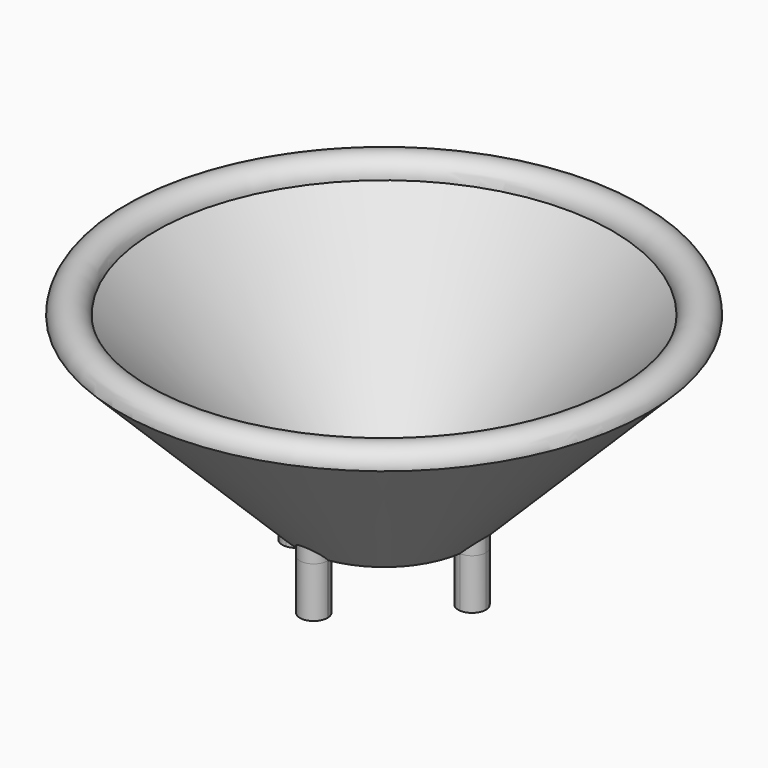
from build123d import *
from build123d import SkipClean  # not in build123d's __all__

# Parameters (mm, degrees)
F4_DEPTH = 10


with BuildPart() as f1:
    # F0 (on Front) → F1 (revolve)
    with BuildSketch(Plane.XZ):
        with BuildLine():
            Line((0, 5), (0, 0))
            Line((0, 0), (17.5, 0))
            Line((17.5, 0), (48.9644660941, 31.4644660941))
            ThreePointArc((48.9644660941, 31.4644660941), (46.4644660941, 32.5), (45.4289321881, 35))
            Line((45.4289321881, 35), (15.4289321881, 5))
            Line((15.4289321881, 5), (0, 5))
        make_face()
        with BuildLine():
            Line((45.4289321881, 35), (52.5, 35))
            ThreePointArc((52.5, 35), (48.9644660941, 38.5355339059), (45.4289321881, 35))
        make_face()
        with BuildLine():
            ThreePointArc((45.4289321881, 35), (46.4644660941, 32.5), (48.9644660941, 31.4644660941))
            Line((48.9644660941, 31.4644660941), (52.5, 35))
            Line((52.5, 35), (45.4289321881, 35))
        make_face()
    revolve(axis=Axis((0, 0, 17.5), (0, 0, 1)))

    # F2 (on face) → F3 (join, up to the next surface of F1)
    with BuildSketch(Plane(origin=(0, 0, 0), x_dir=(1, 0, 0), z_dir=(0, 0, -1))):
        with BuildLine():
            ThreePointArc((17.2839285714, -2.7414983381), (19.3665882743, -2.0194920684), (20.25, 0))
            ThreePointArc((20.25, 0), (19.3665882743, 2.0194920684), (17.2839285714, 2.7414983381))
            ThreePointArc((17.2839285714, 2.7414983381), (17.4458985151, 1.375), (17.5, 0))
            ThreePointArc((17.5, 0), (17.4458985151, -1.375), (17.2839285714, -2.7414983381))
        make_face()
        with BuildLine():
            ThreePointArc((-2.7414983381, 17.2839285714), (0, 17.5), (2.7414983381, 17.2839285714))
            ThreePointArc((2.7414983381, 17.2839285714), (2.7478737625, 17.3918806903), (2.75, 17.5))
            ThreePointArc((2.75, 17.5), (-0.1081193097, 20.2478737625), (-2.7414983381, 17.2839285714))
        make_face()
        with BuildLine():
            ThreePointArc((-2.7414983381, 17.2839285714), (0, 14.75), (2.7414983381, 17.2839285714))
            ThreePointArc((2.7414983381, 17.2839285714), (0, 17.5), (-2.7414983381, 17.2839285714))
        make_face()
        with BuildLine():
            ThreePointArc((2.75, -17.5), (2.7478737625, -17.3918806903), (2.7414983381, -17.2839285714))
            ThreePointArc((2.7414983381, -17.2839285714), (0, -17.5), (-2.7414983381, -17.2839285714))
            ThreePointArc((-2.7414983381, -17.2839285714), (-0.1081193097, -20.2478737625), (2.75, -17.5))
        make_face()
        with BuildLine():
            ThreePointArc((-17.2839285714, -2.7414983381), (-17.5, 0), (-17.2839285714, 2.7414983381))
            ThreePointArc((-17.2839285714, 2.7414983381), (-20.25, 0), (-17.2839285714, -2.7414983381))
        make_face()
    extrude(until=Until.NEXT, dir=(0, 0, 1))

    # F2 (on face) → F4 (join)
    with BuildSketch(Plane(origin=(0, 0, 0), x_dir=(1, 0, 0), z_dir=(0, 0, -1))):
        with BuildLine():
            ThreePointArc((17.2839285714, -2.7414983381), (19.3665882743, -2.0194920684), (20.25, 0))
            ThreePointArc((20.25, 0), (19.3665882743, 2.0194920684), (17.2839285714, 2.7414983381))
            ThreePointArc((17.2839285714, 2.7414983381), (17.4458985151, 1.375), (17.5, 0))
            ThreePointArc((17.5, 0), (17.4458985151, -1.375), (17.2839285714, -2.7414983381))
        make_face()
        with BuildLine():
            ThreePointArc((-2.7414983381, 17.2839285714), (0, 14.75), (2.7414983381, 17.2839285714))
            ThreePointArc((2.7414983381, 17.2839285714), (0, 17.5), (-2.7414983381, 17.2839285714))
        make_face()
        with BuildLine():
            ThreePointArc((-17.2839285714, -2.7414983381), (-17.5, 0), (-17.2839285714, 2.7414983381))
            ThreePointArc((-17.2839285714, 2.7414983381), (-20.25, 0), (-17.2839285714, -2.7414983381))
        make_face()
        with BuildLine():
            ThreePointArc((2.75, -17.5), (2.7478737625, -17.3918806903), (2.7414983381, -17.2839285714))
            ThreePointArc((2.7414983381, -17.2839285714), (0, -17.5), (-2.7414983381, -17.2839285714))
            ThreePointArc((-2.7414983381, -17.2839285714), (-0.1081193097, -20.2478737625), (2.75, -17.5))
        make_face()
        with BuildLine():
            ThreePointArc((-14.75, 0), (-15.4805079316, 1.8665882743), (-17.2839285714, 2.7414983381))
            ThreePointArc((-17.2839285714, 2.7414983381), (-17.5, 0), (-17.2839285714, -2.7414983381))
            ThreePointArc((-17.2839285714, -2.7414983381), (-15.4805079316, -1.8665882743), (-14.75, 0))
        make_face()
        with BuildLine():
            ThreePointArc((-2.7414983381, -17.2839285714), (0, -17.5), (2.7414983381, -17.2839285714))
            ThreePointArc((2.7414983381, -17.2839285714), (0, -14.75), (-2.7414983381, -17.2839285714))
        make_face()
        with BuildLine():
            ThreePointArc((-2.7414983381, 17.2839285714), (0, 17.5), (2.7414983381, 17.2839285714))
            ThreePointArc((2.7414983381, 17.2839285714), (2.7478737625, 17.3918806903), (2.75, 17.5))
            ThreePointArc((2.75, 17.5), (-0.1081193097, 20.2478737625), (-2.7414983381, 17.2839285714))
        make_face()
        with BuildLine():
            ThreePointArc((17.5, 0), (17.4458985151, 1.375), (17.2839285714, 2.7414983381))
            ThreePointArc((17.2839285714, 2.7414983381), (14.75, 0), (17.2839285714, -2.7414983381))
            ThreePointArc((17.2839285714, -2.7414983381), (17.4458985151, -1.375), (17.5, 0))
        make_face()
    with SkipClean():  # cleaning this boolean's faces spoils the solid; the shape is the same uncleaned
        extrude(amount=F4_DEPTH)


solid = f1.part
